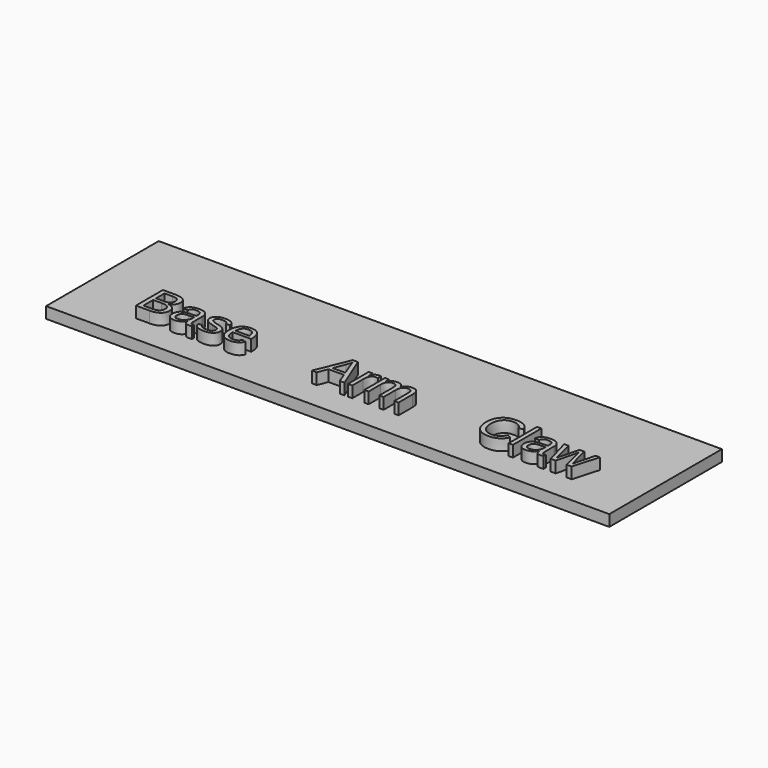
from build123d import *

# Parameters (mm, degrees)
F0_W         = 127
F0_H         = 31.75
F1_DEPTH     = 2.54
F2_TEXT_SIZE = 11.0617015123
F3_DEPTH     = 2.54


# Not quite as in the source:
# - Text() gives the source's letters only with a copy of the font that has no kerning and outlines rounded to 1/6400 em; it was checked with that copy


with BuildPart() as f1:
    # F0 (on Top) → F1 (new body)
    with BuildSketch(Plane.XY):
        with Locations((-1.294657588, 6.6607466385)):
            Rectangle(F0_W, F0_H)
    extrude(amount=F1_DEPTH)

    # F2 (on face) → F3 (join)
    with BuildSketch(Plane.XY.offset(2.54)):
        with Locations((-50.4247694453, -2.9837717234)):
            Text('Base     Arm     Claw', F2_TEXT_SIZE, font='Arimo', text_align=(TextAlign.LEFT, TextAlign.BOTTOM))
    extrude(amount=F3_DEPTH)


solid = f1.part
